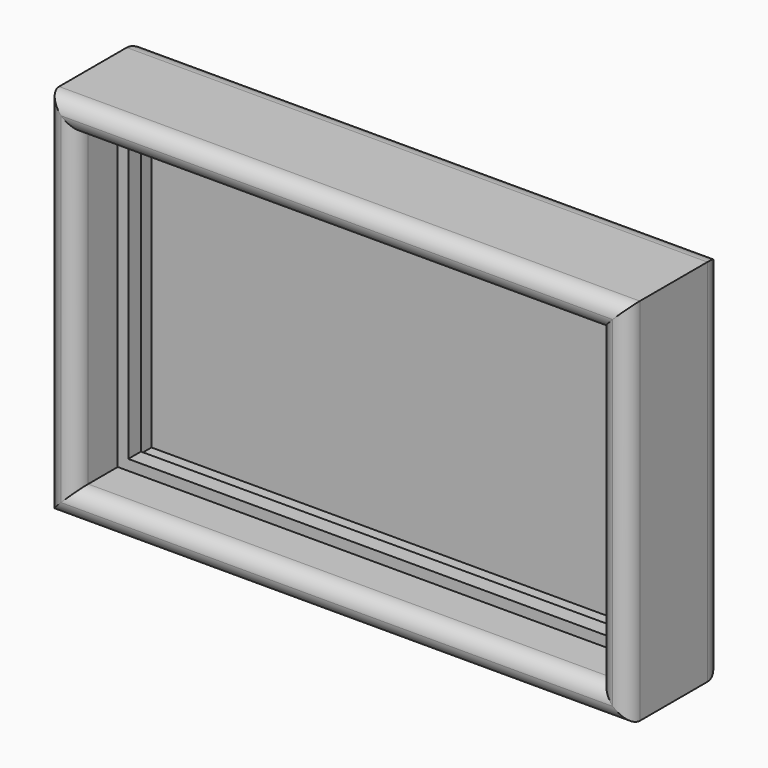
from build123d import *

# Parameters (mm, degrees)
F0_W          = 55
F0_H          = 70
F1_DEPTH      = 10
F2_W          = 99
F2_H          = 59
F3_DEPTH      = 5
F4_W          = 110
F4_H          = 70
F4_W_2        = 99
F4_H_2        = 59
F4_W_3        = 95
F4_H_3        = 55
F5_DEPTH      = 3
F6_W          = 110
F6_H          = 70
F6_W_2        = 99
F6_H_2        = 59
F7_DEPTH      = 10
F8_R          = 4
F9_R          = 3
F10_T1_DEPTH  = 59
F10_T3_DEPTH  = 99
F10_T9_DEPTH  = 106.5
F10_T13_DEPTH = 66.5
F10_T20_DEPTH = 66.5
F10_T24_DEPTH = 106.5
F10_T31_DEPTH = 106.5
F10_T35_DEPTH = 66.5
F10_T42_DEPTH = 106.5
F10_T46_DEPTH = 66.5


# Not quite as in the source:
# - a fillet or chamfer that OpenCascade refuses, or shapes differently, is made with other operations: its cross-section is extruded or revolved along the edge and cut away or added


with BuildPart() as f1:
    # F0 (on Front) → F1 (new body)
    with BuildSketch(Plane.XZ):
        with Locations((-27.5, 0)):
            Rectangle(F0_W, F0_H)
        with Locations((27.5, 0)):
            Rectangle(F0_W, F0_H)
    extrude(amount=F1_DEPTH)

    # F2 (on face) → F3 (cut)
    with BuildSketch(Plane.XZ.offset(10)):
        Rectangle(F2_W, F2_H)
    extrude(amount=-F3_DEPTH, mode=Mode.SUBTRACT)

    # F4 (on face) → F5 (join)
    with BuildSketch(Plane.XZ.offset(10)):
        Rectangle(F4_W, F4_H)
        Rectangle(F4_W_2, F4_H_2, mode=Mode.SUBTRACT)
        Rectangle(F4_W_2, F4_H_2)
        Rectangle(F4_W_3, F4_H_3, mode=Mode.SUBTRACT)
    extrude(amount=F5_DEPTH)

    # F6 (on face) → F7 (join)
    with BuildSketch(Plane.XZ.offset(13)):
        Rectangle(F6_W, F6_H)
        Rectangle(F6_W_2, F6_H_2, mode=Mode.SUBTRACT)
    extrude(amount=F7_DEPTH)

    # F8
    f8_edges = [f1.edges().sort_by_distance(p)[0] for p in [
        (0, 0, 35),
        (-55, 0, 0),
        (55, 0, 0),
        (0, 0, -35),
    ]]
    fillet(f8_edges, radius=F8_R)

    # F9
    f9_edges = [f1.edges().sort_by_distance(p)[0] for p in [
        (-55, -23, 0),
        (0, -23, 35),
        (0, -23, -35),
        (55, -23, 0),
    ]]
    fillet(f9_edges, radius=F9_R)

    # F10: fillet of radius 3 on 4 edges, made by hand

    # F10_s2 → F10_t1 (cut)
    with BuildSketch(Plane.XY.offset(-29.5)):
        with BuildLine():
            ThreePointArc((-52.5, -23), (-50.3786796564, -22.1213203436), (-49.5, -20))
            Line((-49.5, -20), (-49.5, -23))
            Line((-49.5, -23), (-52.5, -23))
        make_face()
        with BuildLine():
            ThreePointArc((52.5, -23), (50.3786796564, -22.1213203436), (49.5, -20))
            Line((49.5, -20), (49.5, -23))
            Line((49.5, -23), (52.5, -23))
        make_face()
    extrude(amount=F10_T1_DEPTH, mode=Mode.SUBTRACT)

    # F10_s4 → F10_t3 (cut)
    with BuildSketch(Plane.YZ.offset(-49.5)):
        with BuildLine():
            ThreePointArc((-23, 32.5), (-22.1213203436, 30.3786796564), (-20, 29.5))
            Line((-20, 29.5), (-23, 29.5))
            Line((-23, 29.5), (-23, 32.5))
        make_face()
        with BuildLine():
            ThreePointArc((-23, -32.5), (-22.1213203436, -30.3786796564), (-20, -29.5))
            Line((-20, -29.5), (-23, -29.5))
            Line((-23, -29.5), (-23, -32.5))
        make_face()
    extrude(amount=F10_T3_DEPTH, mode=Mode.SUBTRACT)


with BuildPart() as f10_tool7:
    # F10_s8 → F10_t9 (new body)
    with BuildSketch(Plane.YZ.offset(49.5)):
        with BuildLine():
            ThreePointArc((-23, -32.5), (-22.1213203436, -30.3786796564), (-20, -29.5))
            Line((-20, -29.5), (-23, -29.5))
            Line((-23, -29.5), (-23, -32.5))
        make_face()
    extrude(amount=-F10_T9_DEPTH)

    split(bisect_by=Plane.YZ.offset(-49.5), keep=Keep.BOTTOM)


with BuildPart() as f10_tool11:
    # F10_s12 → F10_t13 (new body)
    with BuildSketch(Plane.XY.offset(-37)):
        with BuildLine():
            ThreePointArc((-52.5, -23), (-50.3786796564, -22.1213203436), (-49.5, -20))
            Line((-49.5, -20), (-49.5, -23))
            Line((-49.5, -23), (-52.5, -23))
        make_face()
    extrude(amount=F10_T13_DEPTH)

    split(bisect_by=Plane.XY.offset(-29.5), keep=Keep.BOTTOM)


with BuildPart() as f10_tool7_1:
    add(f10_tool7.part)

    # F10_t15: intersect F10_tool11
    add(f10_tool11.part, mode=Mode.INTERSECT)


with BuildPart() as f1_1:
    add(f1.part)

    # F10_t5: cut F10_tool7
    add(f10_tool7_1.part, mode=Mode.SUBTRACT)


with BuildPart() as f10_tool18:
    # F10_s19 → F10_t20 (new body)
    with BuildSketch(Plane.XY.offset(-29.5)):
        with BuildLine():
            ThreePointArc((-52.5, -23), (-50.3786796564, -22.1213203436), (-49.5, -20))
            Line((-49.5, -20), (-49.5, -23))
            Line((-49.5, -23), (-52.5, -23))
        make_face()
    extrude(amount=F10_T20_DEPTH)

    split(bisect_by=Plane.XY.offset(29.5), keep=Keep.TOP)


with BuildPart() as f10_tool22:
    # F10_s23 → F10_t24 (new body)
    with BuildSketch(Plane.YZ.offset(-57)):
        with BuildLine():
            ThreePointArc((-23, 32.5), (-22.1213203436, 30.3786796564), (-20, 29.5))
            Line((-20, 29.5), (-23, 29.5))
            Line((-23, 29.5), (-23, 32.5))
        make_face()
    extrude(amount=F10_T24_DEPTH)

    split(bisect_by=Plane.YZ.offset(-49.5), keep=Keep.BOTTOM)


with BuildPart() as f10_tool18_1:
    add(f10_tool18.part)

    # F10_t26: intersect F10_tool22
    add(f10_tool22.part, mode=Mode.INTERSECT)


with BuildPart() as f1_2:
    add(f1_1.part)

    # F10_t16: cut F10_tool18
    add(f10_tool18_1.part, mode=Mode.SUBTRACT)


with BuildPart() as f10_tool29:
    # F10_s30 → F10_t31 (new body)
    with BuildSketch(Plane.YZ.offset(-49.5)):
        with BuildLine():
            ThreePointArc((-23, 32.5), (-22.1213203436, 30.3786796564), (-20, 29.5))
            Line((-20, 29.5), (-23, 29.5))
            Line((-23, 29.5), (-23, 32.5))
        make_face()
    extrude(amount=F10_T31_DEPTH)

    split(bisect_by=Plane.YZ.offset(49.5), keep=Keep.TOP)


with BuildPart() as f10_tool33:
    # F10_s34 → F10_t35 (new body)
    with BuildSketch(Plane.XY.offset(37)):
        with BuildLine():
            ThreePointArc((52.5, -23), (50.3786796564, -22.1213203436), (49.5, -20))
            Line((49.5, -20), (49.5, -23))
            Line((49.5, -23), (52.5, -23))
        make_face()
    extrude(amount=-F10_T35_DEPTH)

    split(bisect_by=Plane.XY.offset(29.5), keep=Keep.TOP)


with BuildPart() as f10_tool29_1:
    add(f10_tool29.part)

    # F10_t37: intersect F10_tool33
    add(f10_tool33.part, mode=Mode.INTERSECT)


with BuildPart() as f1_3:
    add(f1_2.part)

    # F10_t27: cut F10_tool29
    add(f10_tool29_1.part, mode=Mode.SUBTRACT)


with BuildPart() as f10_tool40:
    # F10_s41 → F10_t42 (new body)
    with BuildSketch(Plane.YZ.offset(57)):
        with BuildLine():
            ThreePointArc((-23, -32.5), (-22.1213203436, -30.3786796564), (-20, -29.5))
            Line((-20, -29.5), (-23, -29.5))
            Line((-23, -29.5), (-23, -32.5))
        make_face()
    extrude(amount=-F10_T42_DEPTH)

    split(bisect_by=Plane.YZ.offset(49.5), keep=Keep.TOP)


with BuildPart() as f10_tool44:
    # F10_s45 → F10_t46 (new body)
    with BuildSketch(Plane.XY.offset(29.5)):
        with BuildLine():
            ThreePointArc((52.5, -23), (50.3786796564, -22.1213203436), (49.5, -20))
            Line((49.5, -20), (49.5, -23))
            Line((49.5, -23), (52.5, -23))
        make_face()
    extrude(amount=-F10_T46_DEPTH)

    split(bisect_by=Plane.XY.offset(-29.5), keep=Keep.BOTTOM)


with BuildPart() as f10_tool40_1:
    add(f10_tool40.part)

    # F10_t48: intersect F10_tool44
    add(f10_tool44.part, mode=Mode.INTERSECT)


with BuildPart() as f1_4:
    add(f1_3.part)

    # F10_t38: cut F10_tool40
    add(f10_tool40_1.part, mode=Mode.SUBTRACT)


solid = f1_4.part
